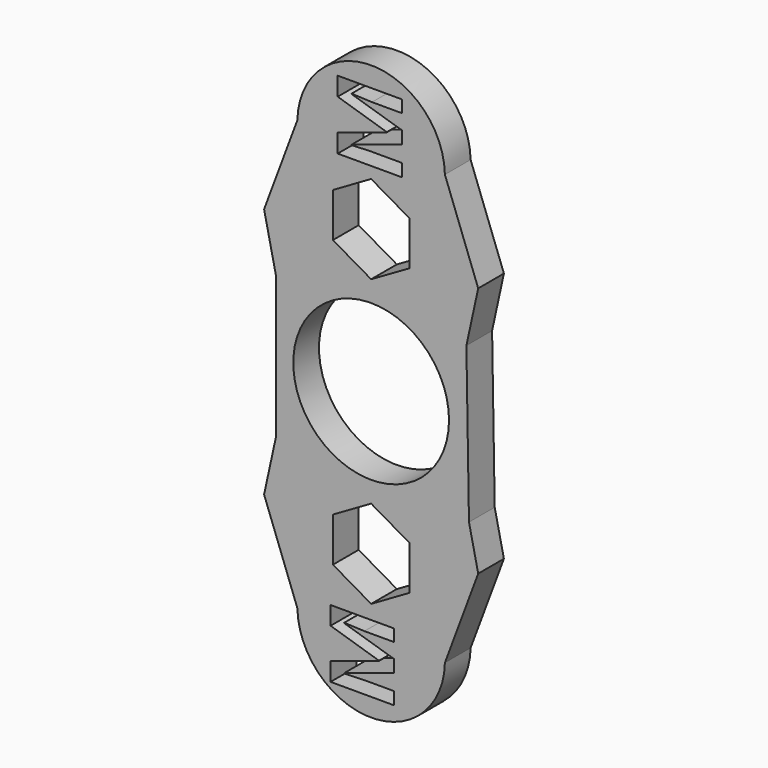
from build123d import *

# Parameters (mm, degrees)
F0_R           = 10.9
F1_DEPTH       = 4.5
F2_TEXT_SIZE   = 12.5849516028
F2_TEXT_SIZE_2 = 12.412709599
F3_DEPTH       = 25


# Not quite as in the source:
# - Text() gives the source's letters only with a copy of the font that has no kerning and outlines rounded to 1/6400 em; it was checked with that copy


with BuildPart() as f1:
    # F0 (on Front) → F1 (new body)
    with BuildSketch(Plane.XZ):
        with BuildLine():
            Line((-14.9855837226, -17.5753161311), (-10.3231193498, -30.0791990012))
            ThreePointArc((-10.3231193498, -30.0791990012), (0, -40.1925636414), (10.3231193498, -30.0791990012))
            Line((10.3231193498, -30.0791990012), (14.9855837226, -17.5753161311))
            Line((14.9855837226, -17.5753161311), (13.6945734564, -11.6507445579))
            Line((13.6945734564, -11.6507445579), (13.3322865657, 9.9881748094))
            Line((13.3322865657, 9.9881748094), (14.9855837226, 17.5753161311))
            Line((14.9855837226, 17.5753161311), (10.3231193498, 30.0791990012))
            ThreePointArc((10.3231193498, 30.0791990012), (0, 40.1925636414), (-10.3231193498, 30.0791990012))
            Line((-10.3231193498, 30.0791990012), (-14.9855837226, 17.5753161311))
            Line((-14.9855837226, 17.5753161311), (-13.3106651756, 9.8889521491))
            Line((-13.3106651756, 9.8889521491), (-13.3106651756, -9.8889521491))
            Line((-13.3106651756, -9.8889521491), (-14.9855837226, -17.5753161311))
        make_face()
        Polygon((0, -26.1776478803), (-5.35, -23.0888239402), (-5.35, -16.9111760598), (0, -13.8223521197), (5.35, -16.9111760598), (5.35, -23.0888239402), align=None, mode=Mode.SUBTRACT)
        Circle(F0_R, mode=Mode.SUBTRACT)
        Polygon((0, 26.1776478803), (5.35, 23.0888239402), (5.35, 16.9111760598), (0, 13.8223521197), (-5.35, 16.9111760598), (-5.35, 23.0888239402), align=None, mode=Mode.SUBTRACT)
    extrude(amount=F1_DEPTH)

    # F2 (on face) → F3 (cut)
    with BuildSketch(Plane(origin=(0, 0, 0), x_dir=(-1, 0, 0), z_dir=(0, 1, 0))):
        with Locations((-23.592489888, -65.5744038522)):
            Text('M', F2_TEXT_SIZE, font='Open Sans', font_style=FontStyle.BOLD, text_align=(TextAlign.LEFT, TextAlign.BOTTOM))
        with Locations(Location((-4.3045146158, 38.5207310319), (0, 0, -90))):
            Text('M', F2_TEXT_SIZE, font='Open Sans', font_style=FontStyle.BOLD, text_align=(TextAlign.LEFT, TextAlign.BOTTOM))
        with Locations(Location((-3.1835793766, -27.0484168406), (0, 0, -90))):
            Text('M', F2_TEXT_SIZE_2, font='Open Sans', font_style=FontStyle.BOLD, text_align=(TextAlign.LEFT, TextAlign.BOTTOM))
    extrude(amount=-F3_DEPTH, mode=Mode.SUBTRACT)


solid = f1.part
